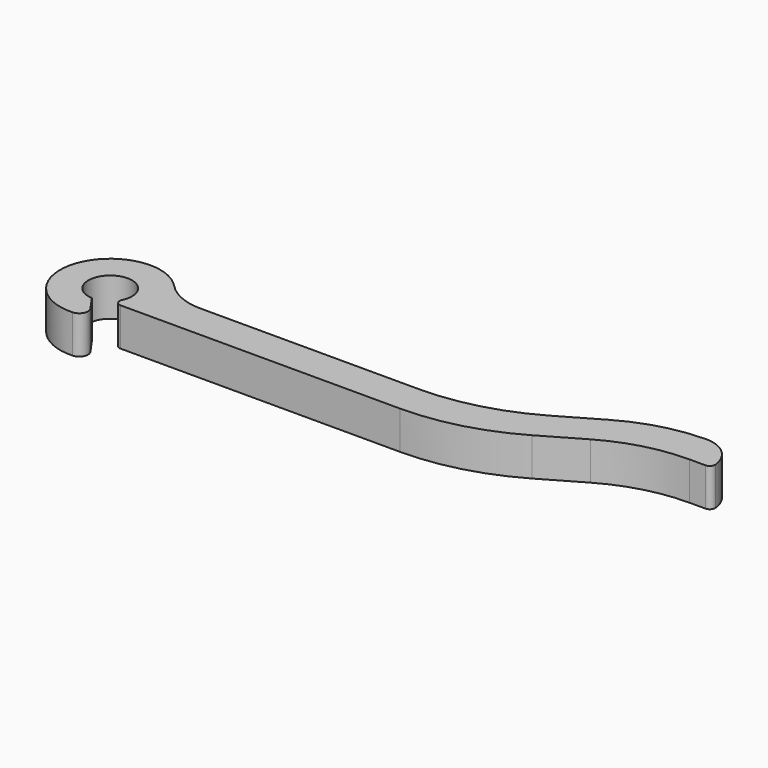
from build123d import *

# Parameters (mm, degrees)
F1_DEPTH = 3.5
F2_R     = 5
F3_R     = 0.8
F4_R     = 3
F5_R     = 0.5


with BuildPart() as f1:
    # F0 (on Top) → F1 (new body)
    with BuildSketch(Plane.XY):
        with BuildLine():
            Line((27.0056332441, 1.6), (4.3127717306, 1.6))
            ThreePointArc((4.3127717306, 1.6), (-4.1689707148, 1.9441407303), (1.5463240937, -4.3323067525))
            Line((1.5463240937, -4.3323067525), (-0.0881351041, -1.9980571072))
            ThreePointArc((-0.0881351041, -1.9980571072), (-1.0206418303, 1.7199680969), (1.7959955457, -0.88))
            ThreePointArc((1.7959955457, -0.88), (1.8207303634, -1.3645751311), (2.2449944321, -1.6))
            Line((2.2449944321, -1.6), (4.3127717306, -1.6))
            Line((4.3127717306, -1.6), (27.8630706599, -1.6))
            ThreePointArc((27.8630706599, -1.6), (33.039451562, -0.9185165258), (37.8630706599, 1.0794919243))
            Line((37.8630706599, 1.0794919243), (41.5192378865, 3.1903810568))
            ThreePointArc((41.5192378865, 3.1903810568), (45.1369522099, 4.6888873943), (49.0192378865, 5.2))
            Line((49.0192378865, 5.2), (51, 5.2))
            Line((51, 5.2), (51, 8.4))
            Line((51, 8.4), (48.1618004707, 8.4))
            ThreePointArc((48.1618004707, 8.4), (44.2795147941, 7.8888873943), (40.6618004707, 6.3903810568))
            Line((40.6618004707, 6.3903810568), (37.0056332441, 4.2794919243))
            ThreePointArc((37.0056332441, 4.2794919243), (32.1820141462, 2.2814834742), (27.0056332441, 1.6))
        make_face()
    extrude(amount=F1_DEPTH)

    # F2
    f2_edges = [f1.edges().sort_by_distance(p)[0] for p in [
        (4.312772, 1.6, 1.75),
        (27.863071, -1.6, 1.75),
    ]]
    fillet(f2_edges, radius=F2_R)

    # F3
    f3_edges = [f1.edges().sort_by_distance(p)[0] for p in [
        (1.546324, -4.332307, 1.75),
    ]]
    fillet(f3_edges, radius=F3_R)

    # F4
    f4_edges = [f1.edges().sort_by_distance(p)[0] for p in [
        (51, 8.4, 1.75),
    ]]
    fillet(f4_edges, radius=F4_R)

    # F5
    f5_edges = [f1.edges().sort_by_distance(p)[0] for p in [
        (51, 5.2, 1.75),
    ]]
    fillet(f5_edges, radius=F5_R)


solid = f1.part
